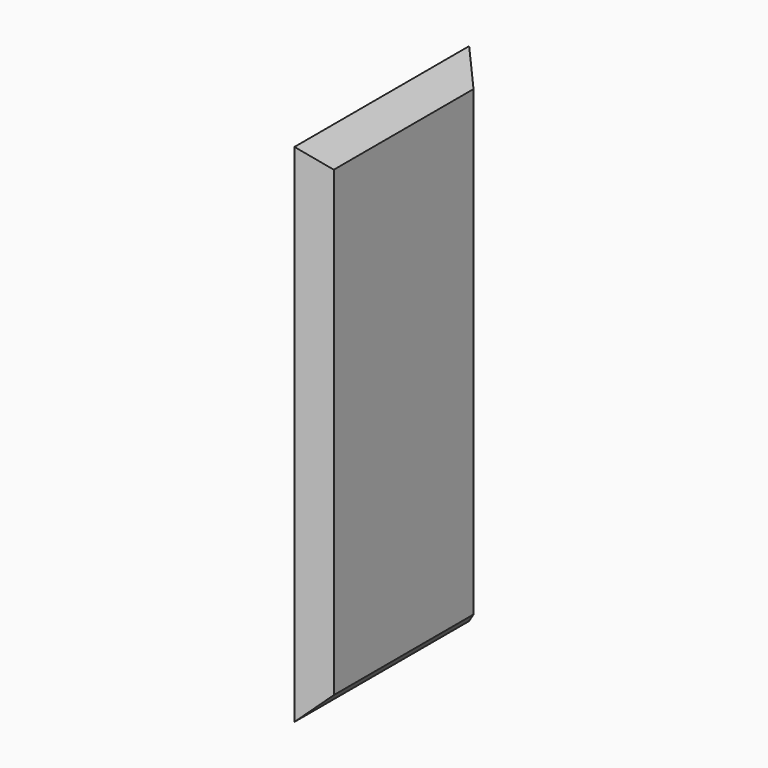
from build123d import *

# Parameters (mm, degrees)
F0_W     = 220
F0_H     = 510
F1_DEPTH = 22
F2_SIZE  = 21.99999


# Not quite as in the source:
# - a fillet or chamfer is up to 0.001 mm smaller than in the source, because OpenCascade refuses the exact size


with BuildPart() as f1:
    # F0 (on Right) → F1 (new body)
    with BuildSketch(Plane.YZ):
        Rectangle(F0_W, F0_H)
    extrude(amount=F1_DEPTH)

    # F2 (size 22 in the source; OpenCascade refuses exactly that, so slightly less here)
    f2_edges = [f1.edges().sort_by_distance(p)[0] for p in [
        (22, 0, 255),
        (22, -110, 0),
        (22, 110, 0),
        (22, 0, -255),
    ]]
    chamfer(f2_edges, length=F2_SIZE)


solid = f1.part
